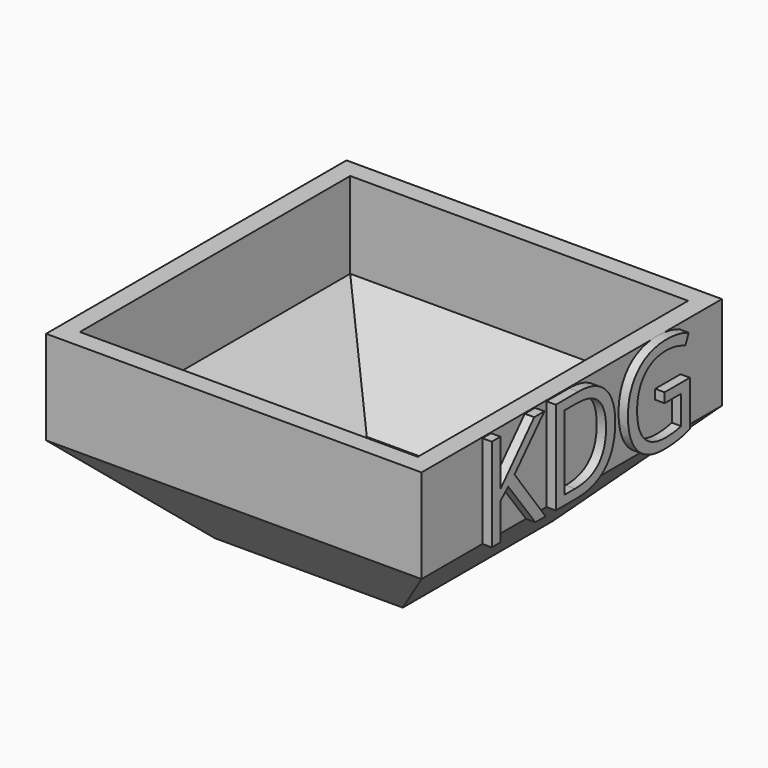
from build123d import *

# Parameters (mm, degrees)
F0_W         = 50.8
F0_H         = 25.4
F1_DEPTH     = 50.8
F2_SIZE      = 12.7
F3_T         = -2.54
F4_TEXT_SIZE = 17.6388888889
F5_DEPTH     = 1.27


# Not quite as in the source:
# - Text() gives the source's letters only with a copy of the font that has no kerning and outlines rounded to 1/6400 em; it was checked with that copy


with BuildPart() as f1:
    # F0 (on Front) → F1 (new body)
    with BuildSketch(Plane.XZ):
        with Locations((-43.7630393267, 20.1818511494)):
            Rectangle(F0_W, F0_H)
    extrude(amount=F1_DEPTH)

    # F2
    f2_edges = [f1.edges().sort_by_distance(p)[0] for p in [
        (-69.163039, -25.4, 7.481851),
        (-18.363039, -25.4, 7.481851),
        (-43.763039, 0, 7.481851),
        (-43.763039, -50.8, 7.481851),
    ]]
    chamfer(f2_edges, length=F2_SIZE)

    # F3
    f3_openings = [f1.faces().sort_by_distance(p)[0] for p in [
        (-43.763039, -25.4, 32.881851),
    ]]
    offset(amount=F3_T, openings=f3_openings)

    # F4 (on face) → F5 (join)
    with BuildSketch(Plane.YZ.offset(-18.3630393267)):
        with Locations((-42.2413051128, 20.1818511494)):
            Text('KDG', F4_TEXT_SIZE, font='Open Sans', text_align=(TextAlign.LEFT, TextAlign.BOTTOM))
    extrude(amount=F5_DEPTH)


solid = f1.part
